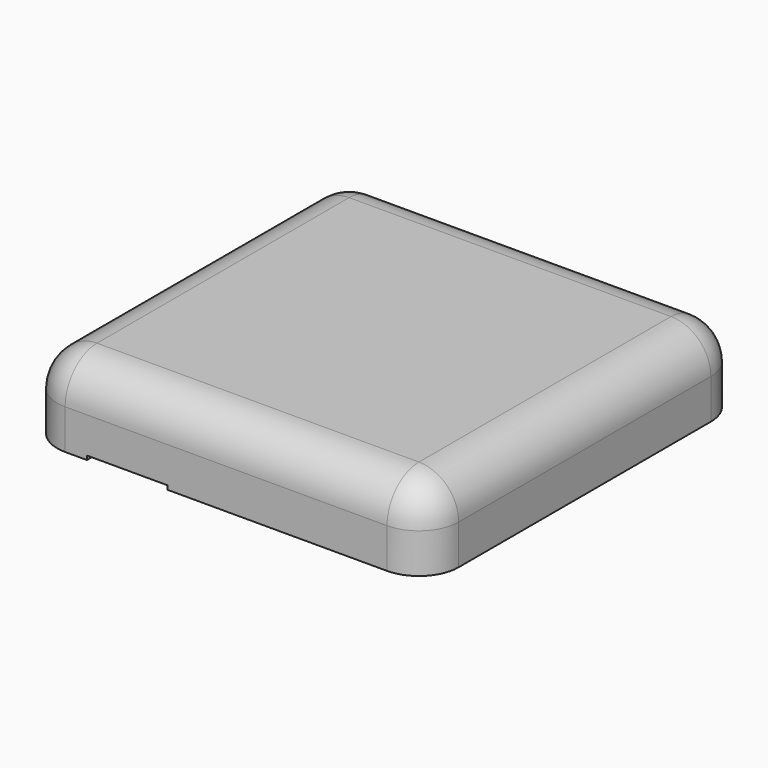
from build123d import *

# Parameters (mm, degrees)
F0_W     = 50.4226610065
F0_H     = 49.5728440583
F1_DEPTH = 10
F2_T     = -5
F3_W     = 10.1061211899
F3_H     = 5
F4_DEPTH = 0.5
F7_D     = 1
F7_DEPTH = 2
F7_TIP   = 0.3004303095
F8_R     = 5
F9_R     = 5


# Not quite as in the source:
# - a feature names something its author has since deleted; it is built from what else it names


with BuildPart() as f1:
    # F0 (on Top) → F1 (new body)
    with BuildSketch(Plane.XY):
        Rectangle(F0_W, F0_H)
    extrude(amount=F1_DEPTH)

    # F2
    f2_openings = [f1.faces().sort_by_distance(p)[0] for p in [
        (0, 0, 0),
    ]]
    offset(amount=F2_T, openings=f2_openings)

    # F3 (on face) → F4 (cut)
    with BuildSketch(Plane(origin=(0, 0, 0), x_dir=(1, 0, 0), z_dir=(0, 0, -1))):
        with Locations((-12.4224121682, 22.2864220291)):
            Rectangle(F3_W, F3_H)
    extrude(amount=-F4_DEPTH, mode=Mode.SUBTRACT)

    # F7
    with Locations(Plane(origin=(0, 0, 0.5), x_dir=(1, 0, 0), z_dir=(0, 0, -1))):
        with Locations((-12.5449625775, 22.3620422184)):
            Hole(F7_D / 2, depth=F7_DEPTH)
            with Locations((0, 0, -(F7_DEPTH + F7_TIP / 2))):  # 118° drill point
                Cone(0, F7_D / 2, F7_TIP, mode=Mode.SUBTRACT)

    # F8
    f8_edges = [f1.edges().sort_by_distance(p)[0] for p in [
        (-25.211331, -24.786422, 5),
        (25.211331, -24.786422, 5),
        (25.211331, 24.786422, 5),
        (-25.211331, 24.786422, 5),
    ]]
    fillet(f8_edges, radius=F8_R)

    # F9
    f9_edges = [f1.edges().sort_by_distance(p)[0] for p in [
        (25.211331, 0, 10),
        (23.746864, -23.321956, 10),
        (23.746864, 23.321956, 10),
        (0, -24.786422, 10),
        (0, 24.786422, 10),
        (-23.746864, -23.321956, 10),
        (-23.746864, 23.321956, 10),
        (-25.211331, 0, 10),
    ]]
    fillet(f9_edges, radius=F9_R)


solid = f1.part
